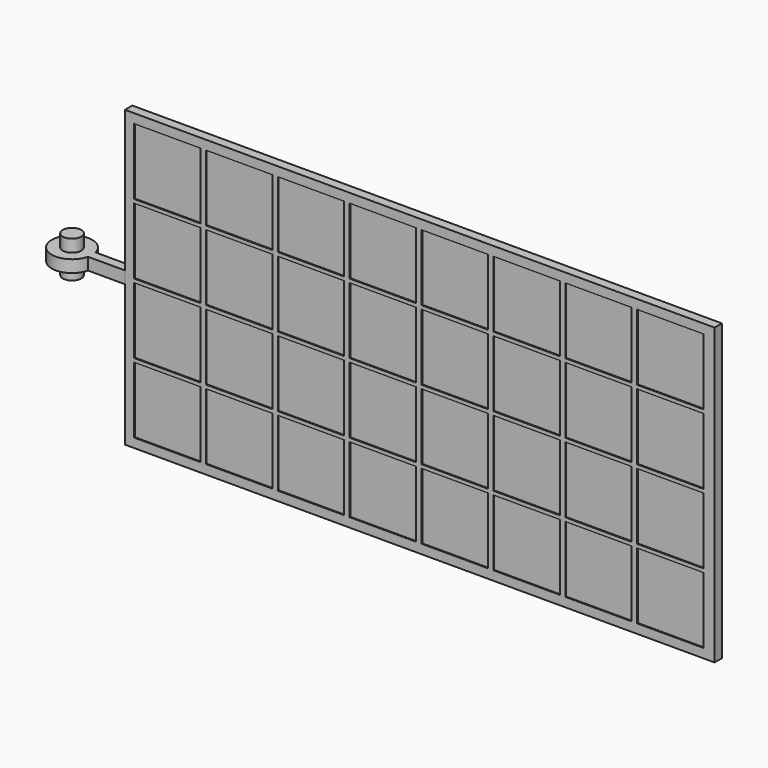
from build123d import *

# Parameters (mm, degrees)
F0_R      = 6.35
F1_DEPTH  = 12.7
F2_R      = 6.35
F3_DEPTH  = 4.191
F4_W      = 45.72
F4_H      = 45.72
F5_DEPTH  = 3.175
F7_W      = 400.05
F7_H      = 196.85
F8_DEPTH  = 2.54
F10_W     = 400.05
F10_H     = 196.85
F11_DEPTH = 5.08


with BuildPart() as f1:
    # F0 (on Top) → F1 (new body, symmetric)
    with BuildSketch(Plane.XY):
        Circle(F0_R)
    extrude(amount=F1_DEPTH, both=True)

    # F2 (on Top) → F3 (join, symmetric)
    with BuildSketch(Plane.XY):
        with BuildLine():
            Line((38.985255793, 3.2560290292), (13.585255793, 3.2560290292))
            ThreePointArc((13.585255793, 3.2560290292), (-13.97, 0), (13.585255793, -3.2560290292))
            Line((13.585255793, -3.2560290292), (38.985255793, -3.2560290292))
            Line((38.985255793, -3.2560290292), (38.985255793, 3.2560290292))
        make_face()
        Circle(F2_R, mode=Mode.SUBTRACT)
    extrude(amount=F3_DEPTH, both=True)

    # F4 (on Front) → F5 (join)
    with BuildSketch(Plane.XZ):
        Polygon((38.985255793, 101.6), (38.985255793, 4.191), (38.985255793, 0), (38.985255793, -4.191), (38.985255793, -101.6), (445.385255793, -101.6), (445.385255793, 101.6), align=None)
        with Locations((68.195255793, -72.39)):
            Rectangle(F4_W, F4_H, mode=Mode.SUBTRACT)
        with Locations((117.725255793, -72.39)):
            Rectangle(F4_W, F4_H, mode=Mode.SUBTRACT)
        with Locations((167.255255793, -72.39)):
            Rectangle(F4_W, F4_H, mode=Mode.SUBTRACT)
        with Locations((216.785255793, -72.39)):
            Rectangle(F4_W, F4_H, mode=Mode.SUBTRACT)
        with Locations((68.195255793, -24.13)):
            Rectangle(F4_W, F4_H, mode=Mode.SUBTRACT)
        with Locations((117.725255793, -24.13)):
            Rectangle(F4_W, F4_H, mode=Mode.SUBTRACT)
        with Locations((167.255255793, -24.13)):
            Rectangle(F4_W, F4_H, mode=Mode.SUBTRACT)
        with Locations((216.785255793, -24.13)):
            Rectangle(F4_W, F4_H, mode=Mode.SUBTRACT)
        with Locations((266.315255793, -72.39)):
            Rectangle(F4_W, F4_H, mode=Mode.SUBTRACT)
        with Locations((315.845255793, -72.39)):
            Rectangle(F4_W, F4_H, mode=Mode.SUBTRACT)
        with Locations((365.375255793, -72.39)):
            Rectangle(F4_W, F4_H, mode=Mode.SUBTRACT)
        with Locations((414.905255793, -72.39)):
            Rectangle(F4_W, F4_H, mode=Mode.SUBTRACT)
        with Locations((266.315255793, -24.13)):
            Rectangle(F4_W, F4_H, mode=Mode.SUBTRACT)
        with Locations((315.845255793, -24.13)):
            Rectangle(F4_W, F4_H, mode=Mode.SUBTRACT)
        with Locations((365.375255793, -24.13)):
            Rectangle(F4_W, F4_H, mode=Mode.SUBTRACT)
        with Locations((414.905255793, -24.13)):
            Rectangle(F4_W, F4_H, mode=Mode.SUBTRACT)
        with Locations((68.195255793, 24.13)):
            Rectangle(F4_W, F4_H, mode=Mode.SUBTRACT)
        with Locations((117.725255793, 24.13)):
            Rectangle(F4_W, F4_H, mode=Mode.SUBTRACT)
        with Locations((167.255255793, 24.13)):
            Rectangle(F4_W, F4_H, mode=Mode.SUBTRACT)
        with Locations((216.785255793, 24.13)):
            Rectangle(F4_W, F4_H, mode=Mode.SUBTRACT)
        with Locations((68.195255793, 72.39)):
            Rectangle(F4_W, F4_H, mode=Mode.SUBTRACT)
        with Locations((117.725255793, 72.39)):
            Rectangle(F4_W, F4_H, mode=Mode.SUBTRACT)
        with Locations((167.255255793, 72.39)):
            Rectangle(F4_W, F4_H, mode=Mode.SUBTRACT)
        with Locations((216.785255793, 72.39)):
            Rectangle(F4_W, F4_H, mode=Mode.SUBTRACT)
        with Locations((266.315255793, 24.13)):
            Rectangle(F4_W, F4_H, mode=Mode.SUBTRACT)
        with Locations((315.845255793, 24.13)):
            Rectangle(F4_W, F4_H, mode=Mode.SUBTRACT)
        with Locations((365.375255793, 24.13)):
            Rectangle(F4_W, F4_H, mode=Mode.SUBTRACT)
        with Locations((414.905255793, 24.13)):
            Rectangle(F4_W, F4_H, mode=Mode.SUBTRACT)
        with Locations((266.315255793, 72.39)):
            Rectangle(F4_W, F4_H, mode=Mode.SUBTRACT)
        with Locations((315.845255793, 72.39)):
            Rectangle(F4_W, F4_H, mode=Mode.SUBTRACT)
        with Locations((365.375255793, 72.39)):
            Rectangle(F4_W, F4_H, mode=Mode.SUBTRACT)
        with Locations((414.905255793, 72.39)):
            Rectangle(F4_W, F4_H, mode=Mode.SUBTRACT)
    extrude(amount=-F5_DEPTH)

    # F7 (on face) → F8 (cut)
    with BuildSketch(Plane.XZ):
        with Locations((241.804255793, 0.381)):
            Rectangle(F7_W, F7_H)
    extrude(amount=-F8_DEPTH, mode=Mode.SUBTRACT)

    # F12: F1 across face


with BuildPart() as f11:
    # F10 (on offset) → F11 (new body)
    with BuildSketch(Plane.XZ.offset(-2.54)):
        with Locations((241.804255793, 0.381)):
            Rectangle(F10_W, F10_H)
    extrude(amount=F11_DEPTH)


with BuildPart() as f1_1:
    add(f1.part)
    add(f1.part.mirror(Plane.XZ))


solid = Compound([f11.part, f1_1.part])
